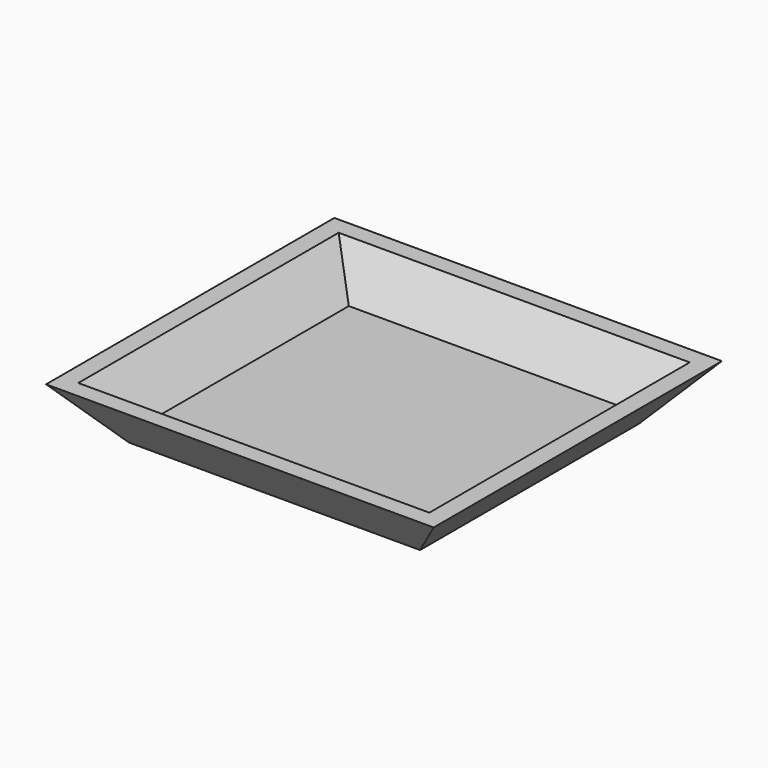
from build123d import *

# Parameters (mm, degrees)
F0_W      = 54.6579919755
F0_H      = 51.4017753303
F1_DEPTH  = 2
F3_W      = 72.7997943759
F3_H      = 67.682877183
F1_FACE_W = 54.6579919755
F1_FACE_H = 51.4017753303
F5_T      = -2.54


# Not quite as in the source:
# - the program builds the solid bodies; features that only make, move or delete a surface that nothing else refers to are left out


with BuildPart() as f1:
    # F0 (on Top) → F1 (new body)
    with BuildSketch(Plane.XY):
        Rectangle(F0_W, F0_H)
    extrude(amount=F1_DEPTH)

    # F3 (on offset) → F4 section 0
    with BuildSketch(Plane.XY.offset(10)):
        Rectangle(F3_W, F3_H)
    # F1_face (on face) → F4 section 1
    with BuildSketch(Plane(origin=(0, 0, 0), x_dir=(1, 0, 0), z_dir=(0, 0, -1))):
        Rectangle(F1_FACE_W, F1_FACE_H)
    loft()

    # F5
    f5_openings = [f1.faces().sort_by_distance(p)[0] for p in [
        (0, 0, 10),
    ]]
    offset(amount=F5_T, openings=f5_openings)


solid = f1.part
